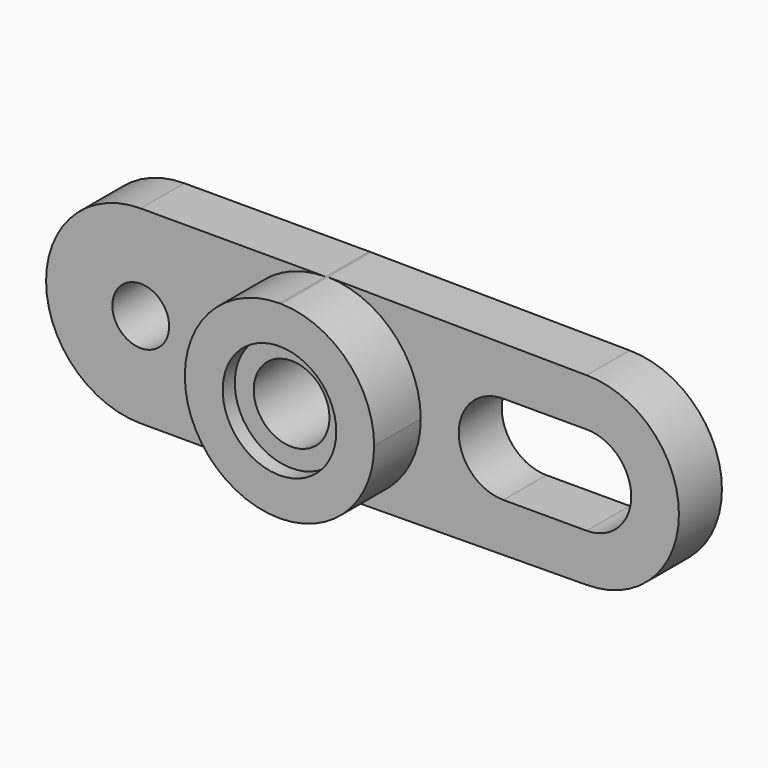
from build123d import *

# Parameters (mm, degrees)
F0_R     = 9.525
F1_DEPTH = 18.288
F0_R_2   = 19.05
F2_DEPTH = 37.592
F3_DEPTH = 18.034
F0_R_3   = 12.7
F5_DEPTH = 32.512


# Not quite as in the source:
# - the program builds the solid bodies; features that only make, move or delete a surface that nothing else refers to are left out


with BuildPart() as f1:
    # F0 (on Front) → F1 (new body)
    with BuildSketch(Plane.XZ):
        with BuildLine():
            ThreePointArc((0, -31.75), (-31.75, 0), (0, 31.75))
            Line((0, 31.75), (-61.9795769453, 31.75))
            ThreePointArc((-61.9795769453, 31.75), (-93.7295769453, 0), (-61.9795769453, -31.75))
            Line((-61.9795769453, -31.75), (0, -31.75))
        make_face()
        with Locations((-61.9795769453, 0)):
            Circle(F0_R, mode=Mode.SUBTRACT)
    extrude(amount=F1_DEPTH)

    # F0 (on Front) → F2 (join)
    with BuildSketch(Plane.XZ):
        with BuildLine():
            Line((0.5778842542, 31.7447405059), (0, 31.75))
            ThreePointArc((0, 31.75), (-31.75, 0), (0, -31.75))
            Line((0, -31.75), (0.5778842542, -31.7447405059))
            ThreePointArc((0.5778842542, -31.7447405059), (22.6540319267, -22.2453891282), (31.75, 0))
            ThreePointArc((31.75, 0), (22.6540319267, 22.2453891282), (0.5778842542, 31.7447405059))
        make_face()
        Circle(F0_R_2, mode=Mode.SUBTRACT)
    extrude(amount=F2_DEPTH)

    # F0 (on Front) → F3 (join)
    with BuildSketch(Plane.XZ):
        with BuildLine():
            Line((87.3840512359, 30.9546921229), (0.5778842542, 31.7447405059))
            ThreePointArc((0.5778842542, 31.7447405059), (22.6540319267, 22.2453891282), (31.75, 0))
            ThreePointArc((31.75, 0), (22.6540319267, -22.2453891282), (0.5778842542, -31.7447405059))
            Line((0.5778842542, -31.7447405059), (87.3840512359, -30.9546921229))
            ThreePointArc((87.3840512359, -30.9546921229), (118.3387433588, 0), (87.3840512359, 30.9546921229))
        make_face()
        with BuildLine():
            ThreePointArc((59.4440512359, -14.9526921229), (44.491359113, 0), (59.4440512359, 14.9526921229))
            Line((59.4440512359, 14.9526921229), (87.3840512359, 14.9526921229))
            ThreePointArc((87.3840512359, 14.9526921229), (102.3367433588, 0), (87.3840512359, -14.9526921229))
            Line((87.3840512359, -14.9526921229), (59.4440512359, -14.9526921229))
        make_face(mode=Mode.SUBTRACT)
    extrude(amount=F3_DEPTH)

    # F0 (on Front) → F5 (join)
    with BuildSketch(Plane.XZ):
        Circle(F0_R_2)
        Circle(F0_R_3, mode=Mode.SUBTRACT)
    extrude(amount=F5_DEPTH)


solid = f1.part
